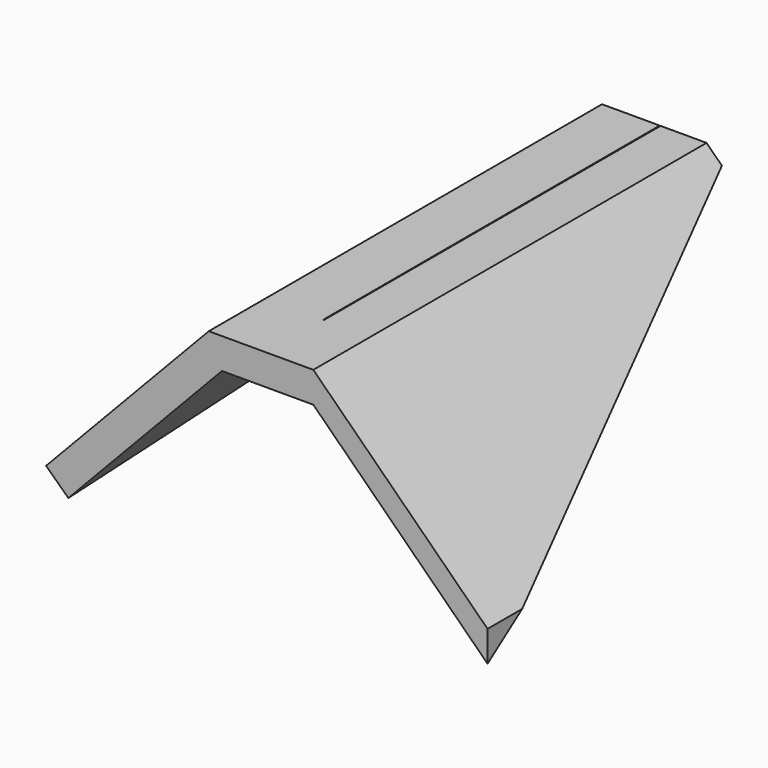
from build123d import *

# Parameters (mm, degrees)
F1_E0_W  = 12.2108995656
F1_E0_H  = 25.4
F2_DEPTH = 1.5875
F1_E1_W  = 5.4040532559
F1_E1_H  = 25.4
F1_E2_W  = 12.6289542233
F1_E2_H  = 25.4
F3_DEPTH = 1.5875
F5_DEPTH = 6.35
F7_DEPTH = 25.4
F9_DEPTH = 3.683


with BuildPart() as f2:
    # F1_E0 (on explicit) → F2 (new body)
    with BuildSketch(Plane(origin=(-11.4085562527, 0, 0), x_dir=(0.6884263284, 0, 0.7253062735), z_dir=(0.7253062735, 0, -0.6884263284))):
        with Locations((6.1054497828, 12.7)):
            Rectangle(F1_E0_W, F1_E0_H)
    extrude(amount=F2_DEPTH)

    # F1_E1 (on explicit) + F1_E2 (on explicit) → F3 (join)
    with BuildSketch(Plane(origin=(-3.0022514984, 0, 8.85664206), x_dir=(1, 0, 0), z_dir=(0, 0, -1))):
        with Locations((2.702026628, 12.7)):
            Rectangle(F1_E1_W, F1_E1_H)
    with BuildSketch(Plane(origin=(2.4018017575, 0, 8.85664206), x_dir=(0.7128696552, 0, -0.7012965526), z_dir=(-0.7012965526, 0, -0.7128696552))):
        with Locations((6.3144771116, 12.7)):
            Rectangle(F1_E2_W, F1_E2_H)
    extrude(amount=F3_DEPTH, dir=(0, 0, -1))

    # F4 (on face) → F5 (cut)
    with BuildSketch(Plane(origin=(-4.850266242, 0, 4.6036427682), x_dir=(0, 1, 0), z_dir=(0.7253062735, 0, -0.6884263284))):
        Polygon((0, 3.6749982582), (-25.4, -7.8539504933), (0, -7.8539504933), align=None)
    extrude(amount=-F5_DEPTH, mode=Mode.SUBTRACT)

    # F6 (on face) → F7 (cut)
    with BuildSketch(Plane(origin=(4.8153308136, 0, 4.8947955096), x_dir=(0.7128696552, 0, -0.7012965526), z_dir=(-0.7012965526, 0, -0.7128696552))):
        Polygon((9.2433015468, 25.4), (-3.3856526765, 0), (9.2433015468, 0), align=None)
    extrude(amount=-F7_DEPTH, mode=Mode.SUBTRACT)

    # F8 (on face) → F9 (cut)
    with BuildSketch(Plane(origin=(0, 0, 8.85664206), x_dir=(1, 0, 0), z_dir=(0, 0, -1))):
        Polygon((0.017724813, 21.7312984169), (-0.0206197838, 21.7312984169), (-0.0206197838, 0), (0.0242347851, 0), align=None)
    extrude(amount=F9_DEPTH, mode=Mode.SUBTRACT)


solid = f2.part
